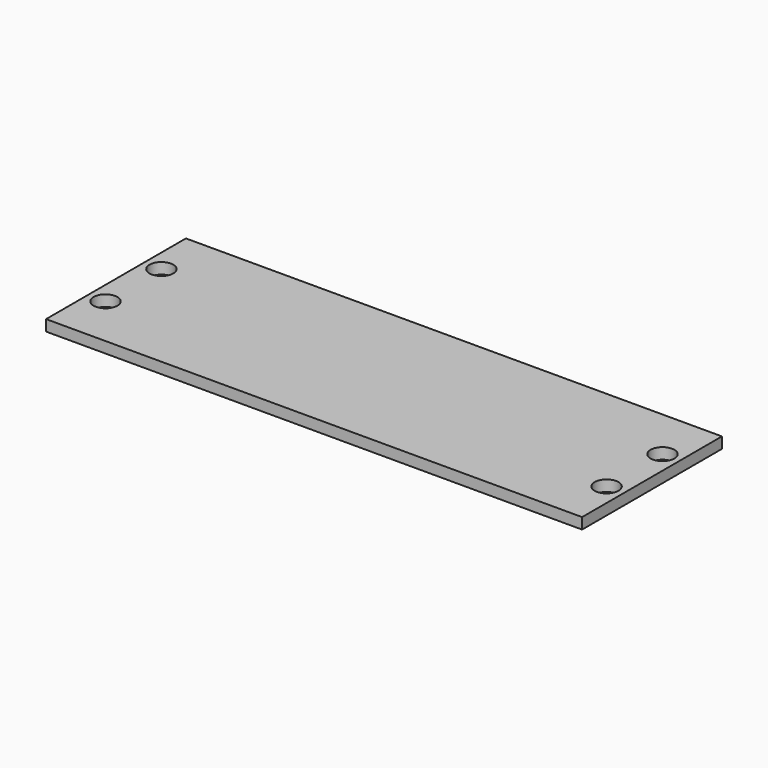
from build123d import *

# Parameters (mm, degrees)
F0_W     = 146.05
F0_H     = 47.625
F0_R     = 3.24
F1_DEPTH = 3


# Not quite as in the source:
# - ends of sketch curves that miss each other by under 0.0002 mm in the source are joined


with BuildPart() as f1:
    # F0 (on Top) → F1 (new body)
    with BuildSketch(Plane.XY):
        Rectangle(F0_W, F0_H)
        with Locations((-68.262, -9.5245)):
            Circle(F0_R, mode=Mode.SUBTRACT)
        with Locations((68.262, -9.5245)):
            Circle(F0_R, mode=Mode.SUBTRACT)
        with Locations((-68.262, 9.5245)):
            Circle(F0_R, mode=Mode.SUBTRACT)
        with BuildLine():
            Line((72.225, -15.859485), (72.225, -23.0125))
            Line((72.225, -23.0125), (-72.225, -23.0125))
            Line((-72.225, -23.0125), (-72.225, -15.874133))
            Line((-72.225, -15.874133), (-68.193705, -15.874133))
            ThreePointArc((-68.193705, -15.874133), (-61.912367271, -9.4562050029), (-68.3302949971, -3.174867271))
            Line((-68.3302949971, -3.174867271), (-72.225, -3.174867))
            Line((-72.225, -3.174867), (-72.225, 3.1745))
            Line((-72.225, 3.1745), (-68.262, 3.1745))
            ThreePointArc((-68.262, 3.1745), (-61.912, 9.5245), (-68.262, 15.8745))
            Line((-68.262, 15.8745), (-72.225, 15.8745))
            Line((-72.225, 15.8745), (-72.225, 23.0125))
            Line((-72.225, 23.0125), (72.225, 23.0125))
            Line((72.225, 23.0125), (72.225, 15.8745))
            Line((72.225, 15.8745), (68.262, 15.8745))
            ThreePointArc((68.262, 15.8745), (61.912, 9.5245), (68.262, 3.1745))
            Line((68.262, 3.1745), (72.225, 3.1745))
            Line((72.225, 3.1745), (72.225, -3.189515))
            Line((72.225, -3.189515), (67.825573, -3.189515))
            ThreePointArc((67.825573, -3.189515), (61.9270152731, -9.9609269812), (68.6984269812, -15.8594847269))
            Line((68.6984269812, -15.8594847269), (72.225, -15.859485))
        make_face(mode=Mode.SUBTRACT)
        with Locations((68.262, 9.5245)):
            Circle(F0_R, mode=Mode.SUBTRACT)
        with BuildLine():
            Line((-72.225, -23.0125), (72.225, -23.0125))
            Line((72.225, -23.0125), (72.225, -15.859485))
            Line((72.225, -15.859485), (68.698427, -15.859485))
            ThreePointArc((68.698427, -15.859485), (61.9270152731, -9.9609269812), (67.8255730188, -3.1895152731))
            Line((67.8255730188, -3.1895152731), (72.225, -3.189515))
            Line((72.225, -3.189515), (72.225, 3.1745))
            Line((72.225, 3.1745), (68.262, 3.1745))
            ThreePointArc((68.262, 3.1745), (61.912, 9.5245), (68.262, 15.8745))
            Line((68.262, 15.8745), (72.225, 15.8745))
            Line((72.225, 15.8745), (72.225, 23.0125))
            Line((72.225, 23.0125), (-72.225, 23.0125))
            Line((-72.225, 23.0125), (-72.225, 15.8745))
            Line((-72.225, 15.8745), (-68.262, 15.8745))
            ThreePointArc((-68.262, 15.8745), (-61.912, 9.5245), (-68.262, 3.1745))
            Line((-68.262, 3.1745), (-72.225, 3.1745))
            Line((-72.225, 3.1745), (-72.225, -3.174867))
            Line((-72.225, -3.174867), (-68.330295, -3.174867))
            ThreePointArc((-68.330295, -3.174867), (-61.912367271, -9.4562050029), (-68.1937050029, -15.874132729))
            Line((-68.1937050029, -15.874132729), (-72.225, -15.874133))
            Line((-72.225, -15.874133), (-72.225, -23.0125))
        make_face()
    extrude(amount=F1_DEPTH)


solid = f1.part
